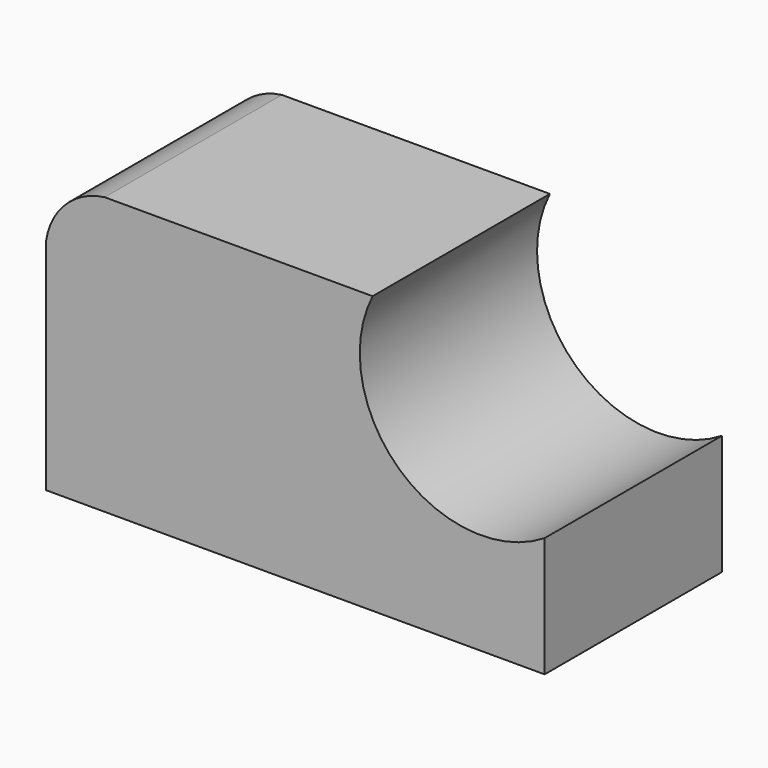
from build123d import *

# Parameters (mm, degrees)
F0_W     = 57.15
F0_H     = 31.75
F1_DEPTH = 25.4
F3_DEPTH = 25.4
F5_R     = 13.8731046092
F6_DEPTH = 25.4


# Not quite as in the source:
# - a feature names something its author has since deleted; it is built from what else it names


with BuildPart() as f1:
    # F0 (on Front) → F1 (new body)
    with BuildSketch(Plane.XZ):
        with Locations((28.575, 15.875)):
            Rectangle(F0_W, F0_H)
    extrude(amount=F1_DEPTH)

    # F2 (on face) → F3 (cut)
    with BuildSketch(Plane.XZ.offset(25.4)):
        with BuildLine():
            ThreePointArc((0, 25.186264758), (2.2625309899, 29.5850653675), (6.7101765828, 31.75))
            Line((6.7101765828, 31.75), (0, 31.75))
            Line((0, 31.75), (0, 25.186264758))
        make_face()
    extrude(amount=-F3_DEPTH, mode=Mode.SUBTRACT)

    # F5 (on face) → F6 (cut)
    with BuildSketch(Plane.XZ.offset(25.4)):
        with Locations((49.8321466148, 25.5351066589)):
            Circle(F5_R)
    extrude(amount=-F6_DEPTH, mode=Mode.SUBTRACT)


solid = f1.part
